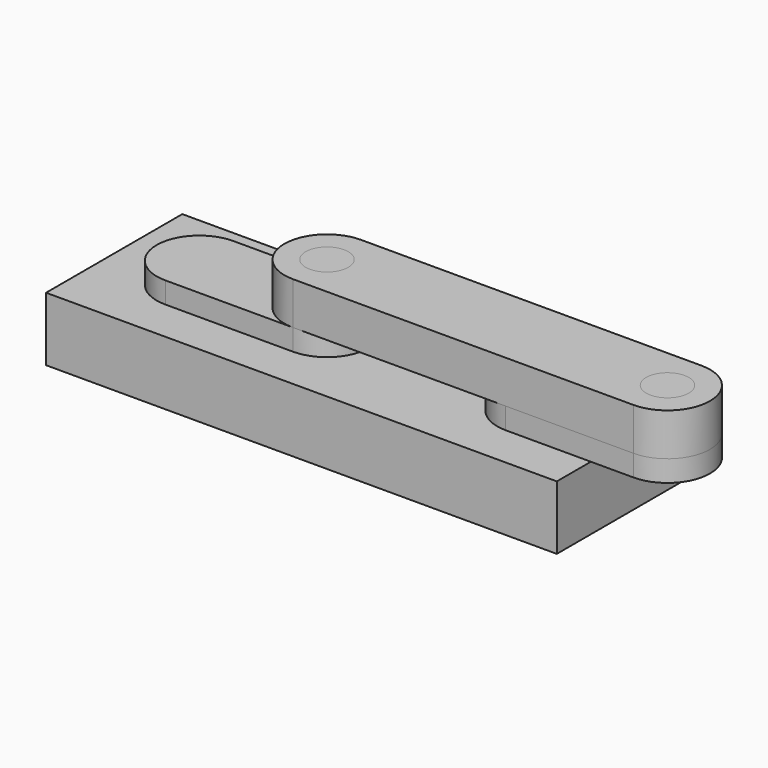
from build123d import *

# Parameters (mm, degrees)
F0_W      = 120
F0_H      = 40
F0_R      = 5
F1_DEPTH  = 15
F4_DEPTH  = 5
F5_R      = 5
F6_DEPTH  = 10
F7_DEPTH  = 15
F8_R      = 5
F9_DEPTH  = 5
F10_R     = 5
F11_DEPTH = 10
F12_DEPTH = 15
F13_R     = 5
F14_DEPTH = 10


with BuildPart() as f1:
    # F0 (on Top) → F1 (new body)
    with BuildSketch(Plane.XY):
        with Locations((60, 20)):
            Rectangle(F0_W, F0_H)
        with Locations((20, 20)):
            Circle(F0_R, mode=Mode.SUBTRACT)
        with Locations((100, 20)):
            Circle(F0_R, mode=Mode.SUBTRACT)
    extrude(amount=F1_DEPTH)


with BuildPart() as f4:
    # F3 (on face) → F4 (new body)
    with BuildSketch(Plane.XY.offset(15)):
        with BuildLine():
            Line((20, 10), (50, 10))
            ThreePointArc((50, 10), (60, 20), (50, 30))
            Line((50, 30), (20, 30))
            ThreePointArc((20, 30), (10, 20), (20, 10))
        make_face()
    extrude(amount=F4_DEPTH)

    # F5 (on face) → F6 (join)
    with BuildSketch(Plane.XY.offset(20)):
        with Locations((50, 20)):
            Circle(F5_R)
    extrude(amount=F6_DEPTH)

    # F0 (on Top) → F7 (join, through all)
    with BuildSketch(Plane.XY):
        with Locations((20, 20)):
            Circle(F0_R)
    extrude(amount=F7_DEPTH)


with BuildPart() as f9:
    # F8 (on face) → F9 (new body)
    with BuildSketch(Plane.XY.offset(15)):
        with BuildLine():
            ThreePointArc((100, 30), (90, 20), (100, 10))
            Line((100, 10), (130, 10))
            ThreePointArc((130, 10), (140, 20), (130, 30))
            Line((130, 30), (100, 30))
        make_face()
        with Locations((100, 20)):
            Circle(F8_R, mode=Mode.SUBTRACT)
        with Locations((100, 20)):
            Circle(F8_R)
    extrude(amount=F9_DEPTH)

    # F10 (on face) → F11 (join)
    with BuildSketch(Plane.XY.offset(20)):
        with Locations((130, 20)):
            Circle(F10_R)
    extrude(amount=F11_DEPTH)


with BuildPart() as f12:
    # F0 (on Top) → F12 (new body, through all)
    with BuildSketch(Plane.XY):
        with Locations((100, 20)):
            Circle(F0_R)
    extrude(amount=F12_DEPTH)


with BuildPart() as f14:
    # F13 (on face) → F14 (new body)
    with BuildSketch(Plane.XY.offset(30)):
        with BuildLine():
            Line((130, 30), (50, 30))
            ThreePointArc((50, 30), (40, 20), (50, 10))
            Line((50, 10), (130, 10))
            ThreePointArc((130, 10), (140, 20), (130, 30))
        make_face()
        with Locations((50, 20)):
            Circle(F13_R, mode=Mode.SUBTRACT)
        with Locations((130, 20)):
            Circle(F13_R, mode=Mode.SUBTRACT)
    extrude(amount=-F14_DEPTH)


solid = Compound([f1.part, f4.part, f9.part, f12.part, f14.part])
